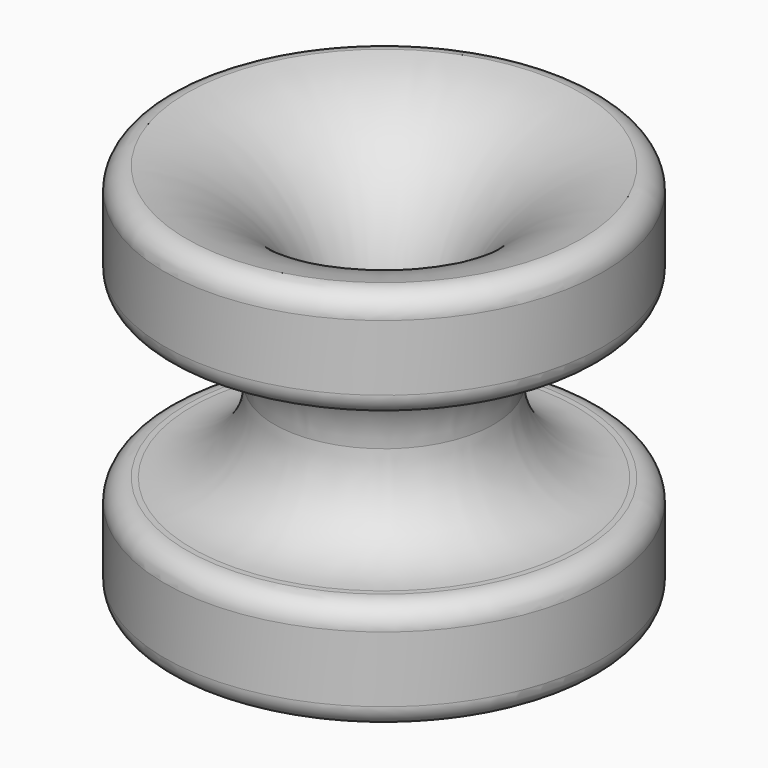
from build123d import *

# Parameters (mm, degrees)
F3_R     = 19.04999
F4_R     = 5.08
F5_R     = 12.7
F6_DEPTH = 88.901


# Not quite as in the source:
# - a variable given as a bare number and used for a length is read in inches; the dataset says mm whatever the document's units were
# - a fillet or chamfer that OpenCascade refuses, or shapes differently, is made with other operations: its cross-section is extruded or revolved along the edge and cut away or added
# - a fillet or chamfer is up to 0.001 mm smaller than in the source, because OpenCascade refuses the exact size


with BuildPart() as f2:
    # F1 (on Front) → F2 (revolve)
    with BuildSketch(Plane.XZ):
        Polygon((0, 44.45), (0, -44.45), (50.8, -44.45), (50.8, -19.05), (25.4, -19.05), (25.4, 0), (25.4, 19.05), (50.8, 19.05), (50.8, 44.45), align=None)
    revolve(axis=Axis((0, 0, 0), (0, 0, 1)))

    # F3 (radius 19.05 in the source; OpenCascade refuses exactly that, so slightly less here)
    f3_edges = [f2.edges().sort_by_distance(p)[0] for p in [
        (-25.4, 0, 19.05),
        (-25.4, 0, -19.05),
    ]]
    fillet(f3_edges, radius=F3_R)

    # F4
    f4_edges = [f2.edges().sort_by_distance(p)[0] for p in [
        (-50.8, 0, 19.05),
        (-50.8, 0, 44.45),
        (-50.8, 0, -44.45),
        (-50.8, 0, -19.05),
    ]]
    fillet(f4_edges, radius=F4_R)

    # F5 (on face) → F6 (cut, through all)
    with BuildSketch(Plane(origin=(0, 0, -44.45), x_dir=(1, 0, 0), z_dir=(0, 0, -1))):
        Circle(F5_R)
    extrude(amount=-F6_DEPTH, mode=Mode.SUBTRACT)

    # F7: fillet of radius 38.1 on 2 edges, made by hand

    # F7_s1 → F7_t2 (revolve, cut)
    with BuildSketch(Plane.XZ):
        with BuildLine():
            ThreePointArc((12.7, 6.6901853818), (22.1193619318, 31.7706758076), (45.72, 44.45))
            Line((45.72, 44.45), (45.6184, 45.2051962924))
            ThreePointArc((45.6184, 45.2051962924), (29.21, 45.212), (12.7, 45.212))
            Line((12.7, 45.212), (11.938, 44.45))
            Line((11.938, 44.45), (11.938, 6.6901853818))
            Line((11.938, 6.6901853818), (12.7, 6.6901853818))
        make_face()
    revolve(axis=Axis((0, 0, 44.45), (0, 0, -1)), mode=Mode.SUBTRACT)

    # F7_s3 → F7_t4 (revolve, cut)
    with BuildSketch(Plane.XZ):
        with BuildLine():
            ThreePointArc((45.72, -44.45), (22.1193619318, -31.7706758076), (12.7, -6.6901853818))
            Line((12.7, -6.6901853818), (11.938, -6.6901853818))
            Line((11.938, -6.6901853818), (11.938, -44.45))
            Line((11.938, -44.45), (12.7, -45.212))
            ThreePointArc((12.7, -45.212), (29.21, -45.212), (45.6184, -45.2051962924))
            Line((45.6184, -45.2051962924), (45.72, -44.45))
        make_face()
    revolve(axis=Axis((0, 0, -44.45), (0, 0, -1)), mode=Mode.SUBTRACT)


solid = f2.part
